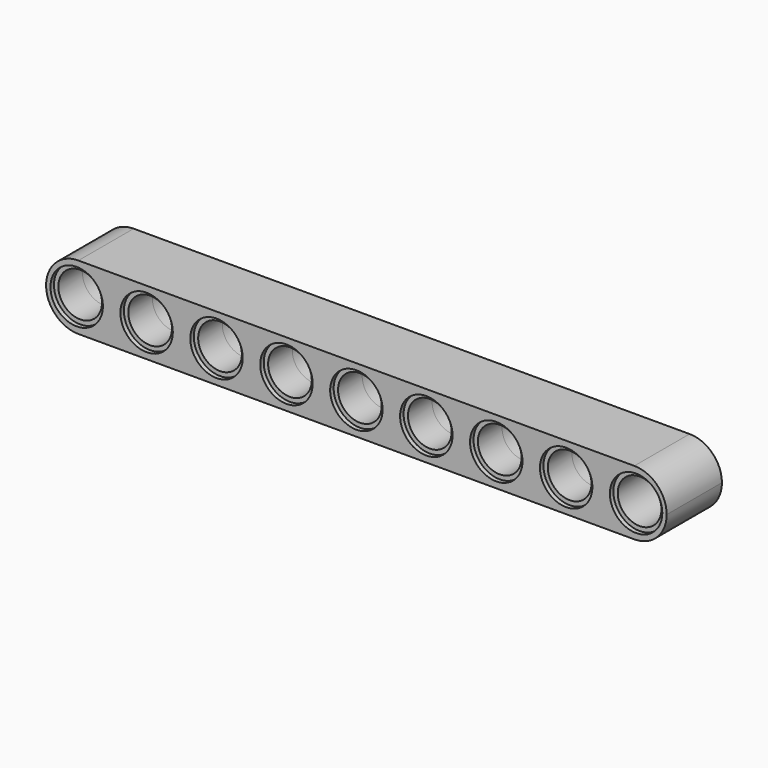
from build123d import *

# Parameters (mm, degrees)
F0_W     = 71
F0_H     = 7.4
F0_R     = 3
F1_DEPTH = 3.95
F0_R_2   = 2.499
F2_DEPTH = 3.45
F3_R     = 3.69999


# Not quite as in the source:
# - a fillet or chamfer is up to 0.001 mm smaller than in the source, because OpenCascade refuses the exact size


with BuildPart() as f1:
    # F0 (on Front) → F1 (new body, symmetric)
    with BuildSketch(Plane.XZ):
        Rectangle(F0_W, F0_H)
        with Locations((-32, 0)):
            Circle(F0_R, mode=Mode.SUBTRACT)
        with Locations((-24, 0)):
            Circle(F0_R, mode=Mode.SUBTRACT)
        with Locations((-16, 0)):
            Circle(F0_R, mode=Mode.SUBTRACT)
        with Locations((-8, 0)):
            Circle(F0_R, mode=Mode.SUBTRACT)
        Circle(F0_R, mode=Mode.SUBTRACT)
        with Locations((8, 0)):
            Circle(F0_R, mode=Mode.SUBTRACT)
        with Locations((16, 0)):
            Circle(F0_R, mode=Mode.SUBTRACT)
        with Locations((24, 0)):
            Circle(F0_R, mode=Mode.SUBTRACT)
        with Locations((32, 0)):
            Circle(F0_R, mode=Mode.SUBTRACT)
    extrude(amount=F1_DEPTH, both=True)

    # F0 (on Front) → F2 (join, symmetric)
    with BuildSketch(Plane.XZ):
        with Locations((-32, 0)):
            Circle(F0_R)
        with Locations((-32, 0)):
            Circle(F0_R_2, mode=Mode.SUBTRACT)
        with Locations((-24, 0)):
            Circle(F0_R)
        with Locations((-24, 0)):
            Circle(F0_R_2, mode=Mode.SUBTRACT)
        with Locations((-16, 0)):
            Circle(F0_R)
        with Locations((-16, 0)):
            Circle(F0_R_2, mode=Mode.SUBTRACT)
        with Locations((-8, 0)):
            Circle(F0_R)
        with Locations((-8, 0)):
            Circle(F0_R_2, mode=Mode.SUBTRACT)
        Circle(F0_R)
        Circle(F0_R_2, mode=Mode.SUBTRACT)
        with Locations((8, 0)):
            Circle(F0_R)
        with Locations((8, 0)):
            Circle(F0_R_2, mode=Mode.SUBTRACT)
        with Locations((16, 0)):
            Circle(F0_R)
        with Locations((16, 0)):
            Circle(F0_R_2, mode=Mode.SUBTRACT)
        with Locations((24, 0)):
            Circle(F0_R)
        with Locations((24, 0)):
            Circle(F0_R_2, mode=Mode.SUBTRACT)
        with Locations((32, 0)):
            Circle(F0_R)
        with Locations((32, 0)):
            Circle(F0_R_2, mode=Mode.SUBTRACT)
    extrude(amount=F2_DEPTH, both=True)

    # F3 (radius 3.7 in the source; OpenCascade refuses exactly that, so slightly less here)
    f3_edges = [f1.edges().sort_by_distance(p)[0] for p in [
        (-35.5, 0, 3.7),
        (-35.5, 0, -3.7),
        (35.5, 0, 3.7),
        (35.5, 0, -3.7),
    ]]
    fillet(f3_edges, radius=F3_R)


solid = f1.part
